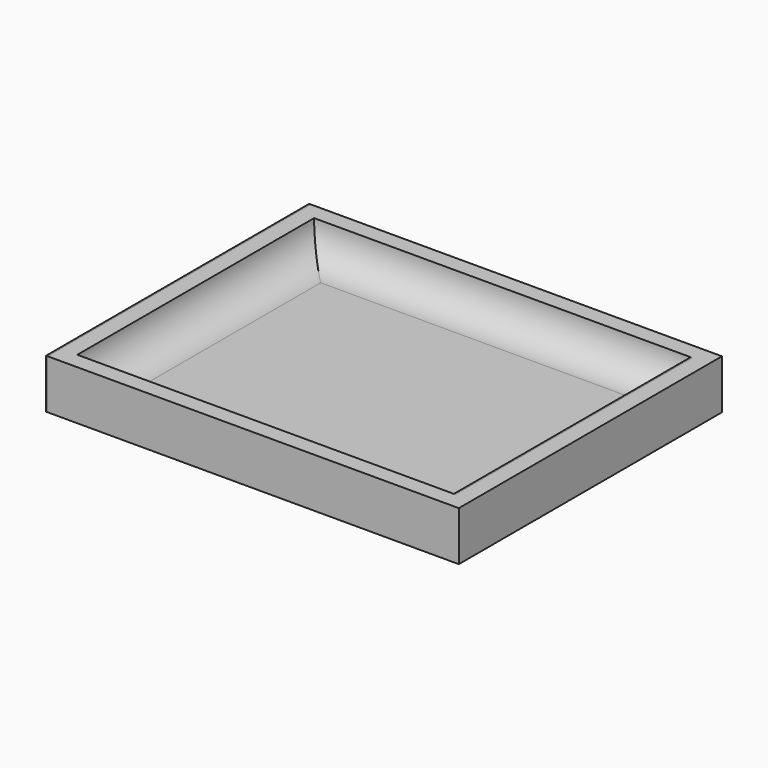
from build123d import *

# Parameters (mm, degrees)
F0_W     = 63.5
F0_H     = 7.62
F1_DEPTH = 25.4
F2_T     = -2.54
F4_R     = 5.07999
F4_2_R   = 5.07999


# Not quite as in the source:
# - a fillet or chamfer is up to 0.001 mm smaller than in the source, because OpenCascade refuses the exact size


with BuildPart() as f1:
    # F0 (on Front) → F1 (new body, symmetric)
    with BuildSketch(Plane.XZ):
        with Locations((-2.1507982165, -11.2475522422)):
            Rectangle(F0_W, F0_H)
    extrude(amount=F1_DEPTH, both=True)

    # F2
    f2_openings = [f1.faces().sort_by_distance(p)[0] for p in [
        (-2.150798, 0, -7.437552),
    ]]
    offset(amount=F2_T, openings=f2_openings)


with BuildPart() as f3_1:
    # F3: copy of F1
    add(f1.part.moved(Location((-0.254, 0, 0))))

    # F4#2 (radius 5.08 in the source; OpenCascade refuses exactly that, so slightly less here)
    f4_2_edges = [f3_1.edges().sort_by_distance(p)[0] for p in [
        (-2.404798, 22.86, -12.517552),
        (26.805202, 0, -12.517552),
    ]]
    fillet(f4_2_edges, radius=F4_2_R)


with BuildPart() as f1_1:
    add(f1.part)

    # F4 (radius 5.08 in the source; OpenCascade refuses exactly that, so slightly less here)
    f4_edges = [f1_1.edges().sort_by_distance(p)[0] for p in [
        (-31.360798, 0, -12.517552),
        (-2.150798, -22.86, -12.517552),
    ]]
    fillet(f4_edges, radius=F4_R)


solid = Compound([f3_1.part, f1_1.part])
